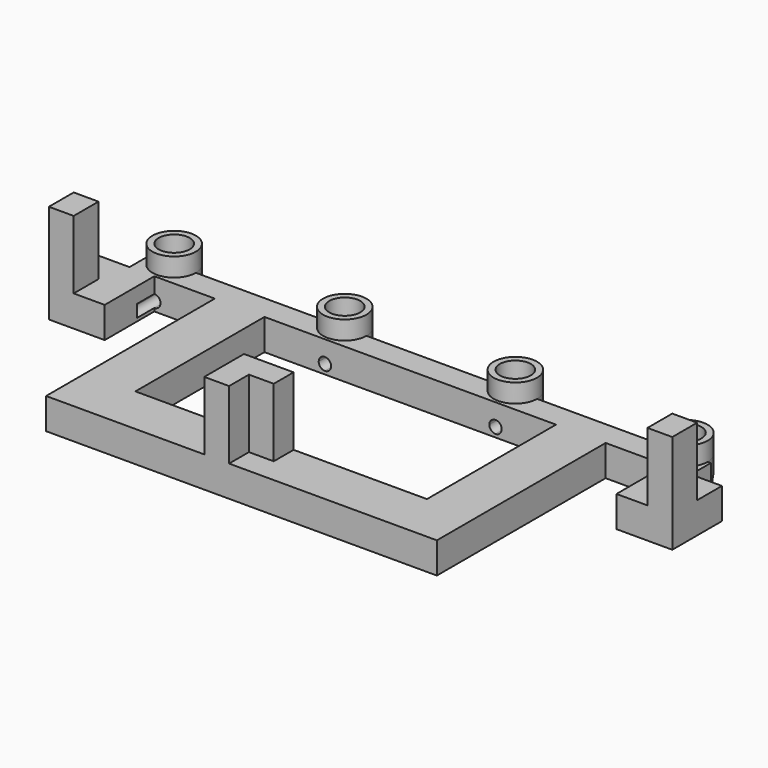
from build123d import *

# Parameters (mm, degrees)
F0_W         = 4
F0_H         = 26
F0_W_2       = 2
F0_H_2       = 4
F0_H_3       = 5
F1_DEPTH     = 5
F2_DEPTH     = 16
F3_R         = 3.5
F3_R_2       = 2.5
F4_DEPTH     = 3
F6_DEPTH     = 7.5
F7_T4_DEPTH  = 26.8255996257
F7_S5_R      = 3.5
F7_T6_DEPTH  = 15
F7_S7_R      = 2.5
F7_T8_DEPTH  = 15
F7_T12_DEPTH = 26.8255996257
F7_S13_R     = 3.5
F7_T14_DEPTH = 15
F7_S15_R     = 2.5
F7_T16_DEPTH = 15
F7_T20_DEPTH = 26.8255996257
F7_S21_R     = 3.5
F7_T22_DEPTH = 15
F7_S23_R     = 2.5
F7_T24_DEPTH = 15
F7_T28_DEPTH = 26.8255996257
F7_S29_R     = 3.5
F7_T30_DEPTH = 15
F7_S31_R     = 2.5
F7_T32_DEPTH = 15
F7_T36_DEPTH = 26.8255996257
F7_S37_R     = 3.5
F7_T38_DEPTH = 15
F7_S39_R     = 2.5
F7_T40_DEPTH = 15
F7_T44_DEPTH = 26.8255996257
F7_S45_R     = 3.5
F7_T46_DEPTH = 15
F7_S47_R     = 2.5
F7_T48_DEPTH = 15
F7_T52_DEPTH = 26.8255996257
F7_S53_R     = 3.5
F7_T54_DEPTH = 15
F7_S55_R     = 2.5
F7_T56_DEPTH = 15
F7_T60_DEPTH = 26.8255996257
F7_S61_R     = 3.5
F7_T62_DEPTH = 15
F7_S63_R     = 2.5
F7_T64_DEPTH = 15


# Not quite as in the source:
# - a fillet or chamfer that OpenCascade refuses, or shapes differently, is made with other operations: its cross-section is extruded or revolved along the edge and cut away or added


with BuildPart() as f1:
    # F0 (on Top) → F1 (new body)
    with BuildSketch(Plane.XY):
        with BuildLine():
            ThreePointArc((27.5, -4), (24.6715728753, -2.8284271247), (23.5, 0))
            Line((23.5, 0), (17.75, 0))
            Line((17.75, 0), (17.75, -4))
            Line((17.75, -4), (27.5, -4))
        make_face()
        with Locations((15.75, -17)):
            Rectangle(F0_W, F0_H)
        with BuildLine():
            Line((52.5, 0), (51, 0))
            ThreePointArc((51, 0), (52.1715728753, -2.8284271247), (55, -4))
            Line((55, -4), (55, -2.5))
            ThreePointArc((55, -2.5), (53.232233047, -1.767766953), (52.5, 0))
        make_face()
        with Locations((42.25, -32)):
            Rectangle(F0_W_2, F0_H_2)
        with BuildLine():
            ThreePointArc((82.5, -2.5), (84.267766953, -1.767766953), (85, 0))
            Line((85, 0), (82.5, 0))
            Line((82.5, 0), (82.5, -2.5))
        make_face()
        with BuildLine():
            Line((82.5, 0), (80, 0))
            ThreePointArc((80, 0), (80.732233047, -1.767766953), (82.5, -2.5))
            Line((82.5, -2.5), (82.5, 0))
        make_face()
        Polygon((47.25, -38), (47.25, -30), (43.25, -30), (43.25, -34), (43.25, -38), align=None)
        with BuildLine():
            Line((64.75, 0), (59, 0))
            ThreePointArc((59, 0), (57.8284271247, -2.8284271247), (55, -4))
            Line((55, -4), (64.75, -4))
            Line((64.75, -4), (64.75, 0))
        make_face()
        with Locations((11.75, -2)):
            Rectangle(F0_W, F0_H_2)
        with Locations((42.25, -36)):
            Rectangle(F0_W_2, F0_H_2)
        with Locations((40.25, -32)):
            Rectangle(F0_W_2, F0_H_2)
        with Locations((11.75, -17)):
            Rectangle(F0_W, F0_H)
        with Locations((70.75, -2)):
            Rectangle(F0_W, F0_H_2)
        with BuildLine():
            Line((25, 0), (23.5, 0))
            ThreePointArc((23.5, 0), (24.6715728753, -2.8284271247), (27.5, -4))
            Line((27.5, -4), (27.5, -2.5))
            ThreePointArc((27.5, -2.5), (25.732233047, -1.767766953), (25, 0))
        make_face()
        with Locations((40.25, -36)):
            Rectangle(F0_W_2, F0_H_2)
        Polygon((35.25, -30), (35.25, -38), (39.25, -38), (39.25, -34), (39.25, -30), align=None)
        with BuildLine():
            ThreePointArc((55, -4), (57.8284271247, -2.8284271247), (59, 0))
            Line((59, 0), (57.5, 0))
            ThreePointArc((57.5, 0), (56.767766953, -1.767766953), (55, -2.5))
            Line((55, -2.5), (55, -4))
        make_face()
        with Locations((70.75, -17)):
            Rectangle(F0_W, F0_H)
        with Locations((66.75, -2)):
            Rectangle(F0_W, F0_H_2)
        with BuildLine():
            Line((55, 0), (52.5, 0))
            ThreePointArc((52.5, 0), (53.232233047, -1.767766953), (55, -2.5))
            Line((55, -2.5), (55, 0))
        make_face()
        with BuildLine():
            Line((0, -4), (0, -2.5))
            ThreePointArc((0, -2.5), (-1.767766953, -1.767766953), (-2.5, 0))
            Line((-2.5, 0), (-4, 0))
            ThreePointArc((-4, 0), (-2.8284271247, -2.8284271247), (0, -4))
        make_face()
        Polygon((86.5, -4), (82.5, -4), (82.5, -14), (87.5, -14), (87.5, -9), (87.5, -4), align=None)
        with BuildLine():
            Line((-4, -4), (0, -4))
            ThreePointArc((0, -4), (-2.8284271247, -2.8284271247), (-4, 0))
            Line((-4, 0), (-4, -4))
        make_face()
        with BuildLine():
            Line((86.5, -4), (86.5, 0))
            ThreePointArc((86.5, 0), (85.3284271247, -2.8284271247), (82.5, -4))
            Line((82.5, -4), (86.5, -4))
        make_face()
        with Locations((-7, -6.5)):
            Rectangle(F0_W, F0_H_3)
        with Locations((89.5, -6.5)):
            Rectangle(F0_W, F0_H_3)
        with Locations((-7, -11.5)):
            Rectangle(F0_W, F0_H_3)
        with Locations((89.5, -11.5)):
            Rectangle(F0_W, F0_H_3)
        with BuildLine():
            Line((2.5, 0), (0, 0))
            Line((0, 0), (0, -2.5))
            ThreePointArc((0, -2.5), (1.767766953, -1.767766953), (2.5, 0))
        make_face()
        with BuildLine():
            Line((9.75, 0), (4, 0))
            ThreePointArc((4, 0), (2.8284271247, -2.8284271247), (0, -4))
            Line((0, -4), (9.75, -4))
            Line((9.75, -4), (9.75, 0))
        make_face()
        with BuildLine():
            Line((27.5, 0), (25, 0))
            ThreePointArc((25, 0), (25.732233047, -1.767766953), (27.5, -2.5))
            Line((27.5, -2.5), (27.5, 0))
        make_face()
        with BuildLine():
            ThreePointArc((27.5, -2.5), (29.267766953, -1.767766953), (30, 0))
            Line((30, 0), (27.5, 0))
            Line((27.5, 0), (27.5, -2.5))
        make_face()
        with Locations((66.75, -17)):
            Rectangle(F0_W, F0_H)
        with BuildLine():
            ThreePointArc((27.5, -4), (30.3284271247, -2.8284271247), (31.5, 0))
            Line((31.5, 0), (30, 0))
            ThreePointArc((30, 0), (29.267766953, -1.767766953), (27.5, -2.5))
            Line((27.5, -2.5), (27.5, -4))
        make_face()
        with BuildLine():
            Line((0, -2.5), (0, 0))
            Line((0, 0), (-2.5, 0))
            ThreePointArc((-2.5, 0), (-1.767766953, -1.767766953), (0, -2.5))
        make_face()
        with BuildLine():
            ThreePointArc((55, -2.5), (56.767766953, -1.767766953), (57.5, 0))
            Line((57.5, 0), (55, 0))
            Line((55, 0), (55, -2.5))
        make_face()
        with BuildLine():
            ThreePointArc((82.5, -4), (85.3284271247, -2.8284271247), (86.5, 0))
            Line((86.5, 0), (85, 0))
            ThreePointArc((85, 0), (84.267766953, -1.767766953), (82.5, -2.5))
            Line((82.5, -2.5), (82.5, -4))
        make_face()
        Polygon((13.75, -30), (9.75, -30), (9.75, -38), (35.25, -38), (35.25, -30), (17.75, -30), align=None)
        with BuildLine():
            Line((51, 0), (31.5, 0))
            ThreePointArc((31.5, 0), (30.3284271247, -2.8284271247), (27.5, -4))
            Line((27.5, -4), (55, -4))
            ThreePointArc((55, -4), (52.1715728753, -2.8284271247), (51, 0))
        make_face()
        with BuildLine():
            ThreePointArc((82.5, -4), (79.6715728753, -2.8284271247), (78.5, 0))
            Line((78.5, 0), (72.75, 0))
            Line((72.75, 0), (72.75, -4))
            Line((72.75, -4), (82.5, -4))
        make_face()
        with Locations((15.75, -2)):
            Rectangle(F0_W, F0_H_2)
        with BuildLine():
            Line((4, 0), (2.5, 0))
            ThreePointArc((2.5, 0), (1.767766953, -1.767766953), (0, -2.5))
            Line((0, -2.5), (0, -4))
            ThreePointArc((0, -4), (2.8284271247, -2.8284271247), (4, 0))
        make_face()
        Polygon((68.75, -30), (64.75, -30), (47.25, -30), (47.25, -38), (72.75, -38), (72.75, -30), align=None)
        Polygon((0, -14), (0, -4), (-4, -4), (-5, -4), (-5, -9), (-5, -14), align=None)
        with BuildLine():
            Line((80, 0), (78.5, 0))
            ThreePointArc((78.5, 0), (79.6715728753, -2.8284271247), (82.5, -4))
            Line((82.5, -4), (82.5, -2.5))
            ThreePointArc((82.5, -2.5), (80.732233047, -1.767766953), (80, 0))
        make_face()
    extrude(amount=F1_DEPTH)

    # F0 (on Top) → F2 (join)
    with BuildSketch(Plane.XY):
        with Locations((-7, -11.5)):
            Rectangle(F0_W, F0_H_3)
        with Locations((89.5, -11.5)):
            Rectangle(F0_W, F0_H_3)
        Polygon((35.25, -30), (35.25, -38), (39.25, -38), (39.25, -34), (39.25, -30), align=None)
        with Locations((40.25, -32)):
            Rectangle(F0_W_2, F0_H_2)
        with Locations((42.25, -32)):
            Rectangle(F0_W_2, F0_H_2)
    extrude(amount=F2_DEPTH)

    # F3 (on face) → F4 (join)
    with BuildSketch(Plane.XY.offset(5)):
        Circle(F3_R)
        Circle(F3_R_2, mode=Mode.SUBTRACT)
        with BuildLine():
            ThreePointArc((86, 0), (82.5, 3.5), (79, 0))
            ThreePointArc((79, 0), (82.5, -3.5), (86, 0))
        make_face()
        with BuildLine():
            ThreePointArc((85, 0), (82.5, -2.5), (80, 0))
            ThreePointArc((80, 0), (82.5, 2.5), (85, 0))
        make_face(mode=Mode.SUBTRACT)
        with BuildLine():
            ThreePointArc((58.5, 0), (55, 3.5), (51.5, 0))
            Line((51.5, 0), (52.5, 0))
            ThreePointArc((52.5, 0), (55, 2.5), (57.5, 0))
            Line((57.5, 0), (58.5, 0))
        make_face()
        with BuildLine():
            Line((52.5, 0), (51.5, 0))
            ThreePointArc((51.5, 0), (55, -3.5), (58.5, 0))
            Line((58.5, 0), (57.5, 0))
            ThreePointArc((57.5, 0), (55, -2.5), (52.5, 0))
        make_face()
        with BuildLine():
            ThreePointArc((31, 0), (27.5, 3.5), (24, 0))
            Line((24, 0), (25, 0))
            ThreePointArc((25, 0), (27.5, 2.5), (30, 0))
            Line((30, 0), (31, 0))
        make_face()
        with BuildLine():
            Line((25, 0), (24, 0))
            ThreePointArc((24, 0), (27.5, -3.5), (31, 0))
            Line((31, 0), (30, 0))
            ThreePointArc((30, 0), (27.5, -2.5), (25, 0))
        make_face()
    extrude(amount=F4_DEPTH)

    # F5 (on face) → F6 (cut)
    with BuildSketch(Plane(origin=(0, 0, 0), x_dir=(-1, 0, 0), z_dir=(0, 1, 0))):
        with BuildLine():
            ThreePointArc((0, 2.5), (-1, 1.5), (0, 0.5))
            Line((0, 0.5), (0, 2.5))
        make_face()
        with BuildLine():
            Line((0, 2.5), (0, 0.5))
            ThreePointArc((0, 0.5), (0.7071067812, 0.7928932188), (1, 1.5))
            ThreePointArc((1, 1.5), (0.7071067812, 2.2071067812), (0, 2.5))
        make_face()
        with BuildLine():
            ThreePointArc((-82.5, 2.5), (-83.5, 1.5), (-82.5, 0.5))
            Line((-82.5, 0.5), (-82.5, 2.5))
        make_face()
        with BuildLine():
            Line((-82.5, 2.5), (-82.5, 0.5))
            ThreePointArc((-82.5, 0.5), (-81.7928932188, 0.7928932188), (-81.5, 1.5))
            ThreePointArc((-81.5, 1.5), (-81.7928932188, 2.2071067812), (-82.5, 2.5))
        make_face()
        with BuildLine():
            ThreePointArc((-55, 2.5), (-56, 1.5), (-55, 0.5))
            Line((-55, 0.5), (-55, 2.5))
        make_face()
        with BuildLine():
            Line((-55, 2.5), (-55, 0.5))
            ThreePointArc((-55, 0.5), (-54.2928932188, 0.7928932188), (-54, 1.5))
            ThreePointArc((-54, 1.5), (-54.2928932188, 2.2071067812), (-55, 2.5))
        make_face()
        with BuildLine():
            ThreePointArc((-27.5, 2.5), (-28.5, 1.5), (-27.5, 0.5))
            Line((-27.5, 0.5), (-27.5, 2.5))
        make_face()
        with BuildLine():
            Line((-27.5, 2.5), (-27.5, 0.5))
            ThreePointArc((-27.5, 0.5), (-26.7928932188, 0.7928932188), (-26.5, 1.5))
            ThreePointArc((-26.5, 1.5), (-26.7928932188, 2.2071067812), (-27.5, 2.5))
        make_face()
    extrude(amount=-F6_DEPTH, mode=Mode.SUBTRACT)

    # F7: chamfer of 5 x 3.5 on 8 edges, made by hand


with BuildPart() as f7_tool2:
    # F7_s3 → F7_t4 (new body)
    with BuildSketch(Plane.YZ.offset(16.4127998128)):
        Polygon((0, 0), (3.5, 5), (0, 5), align=None)
    extrude(amount=-F7_T4_DEPTH)

    # F7_s5 → F7_t6 (intersect, symmetric)
    with BuildSketch(Plane.XY.offset(2.5)):
        Circle(F7_S5_R)
    extrude(amount=F7_T6_DEPTH, both=True, mode=Mode.INTERSECT)

    # F7_s7 → F7_t8 (cut, symmetric)
    with BuildSketch(Plane.XY.offset(2.5)):
        Circle(F7_S7_R)
    extrude(amount=F7_T8_DEPTH, both=True, mode=Mode.SUBTRACT)


with BuildPart() as f1_1:
    add(f1.part)

    # F7_t1: union F7_tool2
    add(f7_tool2.part)


with BuildPart() as f7_tool10:
    # F7_s11 → F7_t12 (new body)
    with BuildSketch(Plane.YZ.offset(37.9127998128)):
        Polygon((0, 0), (3.5, 5), (0, 5), align=None)
    extrude(amount=-F7_T12_DEPTH)

    # F7_s13 → F7_t14 (intersect, symmetric)
    with BuildSketch(Plane.XY.offset(2.5)):
        with Locations((27.5, 0)):
            Circle(F7_S13_R)
    extrude(amount=F7_T14_DEPTH, both=True, mode=Mode.INTERSECT)

    # F7_s15 → F7_t16 (cut, symmetric)
    with BuildSketch(Plane.XY.offset(2.5)):
        with Locations((27.5, 0)):
            Circle(F7_S15_R)
    extrude(amount=F7_T16_DEPTH, both=True, mode=Mode.SUBTRACT)


with BuildPart() as f1_2:
    add(f1_1.part)

    # F7_t9: union F7_tool10
    add(f7_tool10.part)


with BuildPart() as f7_tool18:
    # F7_s19 → F7_t20 (new body)
    with BuildSketch(Plane.YZ.offset(65.4127998128)):
        Polygon((0, 0), (3.5, 5), (0, 5), align=None)
    extrude(amount=-F7_T20_DEPTH)

    # F7_s21 → F7_t22 (intersect, symmetric)
    with BuildSketch(Plane.XY.offset(2.5)):
        with Locations((55, 0)):
            Circle(F7_S21_R)
    extrude(amount=F7_T22_DEPTH, both=True, mode=Mode.INTERSECT)

    # F7_s23 → F7_t24 (cut, symmetric)
    with BuildSketch(Plane.XY.offset(2.5)):
        with Locations((55, 0)):
            Circle(F7_S23_R)
    extrude(amount=F7_T24_DEPTH, both=True, mode=Mode.SUBTRACT)


with BuildPart() as f1_3:
    add(f1_2.part)

    # F7_t17: union F7_tool18
    add(f7_tool18.part)


with BuildPart() as f7_tool26:
    # F7_s27 → F7_t28 (new body)
    with BuildSketch(Plane.YZ.offset(43.9127998128)):
        Polygon((0, 0), (3.5, 5), (0, 5), align=None)
    extrude(amount=-F7_T28_DEPTH)

    # F7_s29 → F7_t30 (intersect, symmetric)
    with BuildSketch(Plane.XY.offset(2.5)):
        with Locations((27.5, 0)):
            Circle(F7_S29_R)
    extrude(amount=F7_T30_DEPTH, both=True, mode=Mode.INTERSECT)

    # F7_s31 → F7_t32 (cut, symmetric)
    with BuildSketch(Plane.XY.offset(2.5)):
        with Locations((27.5, 0)):
            Circle(F7_S31_R)
    extrude(amount=F7_T32_DEPTH, both=True, mode=Mode.SUBTRACT)


with BuildPart() as f1_4:
    add(f1_3.part)

    # F7_t25: union F7_tool26
    add(f7_tool26.part)


with BuildPart() as f7_tool34:
    # F7_s35 → F7_t36 (new body)
    with BuildSketch(Plane.YZ.offset(92.9127998128)):
        Polygon((0, 0), (3.5, 5), (0, 5), align=None)
    extrude(amount=-F7_T36_DEPTH)

    # F7_s37 → F7_t38 (intersect, symmetric)
    with BuildSketch(Plane.XY.offset(2.5)):
        with Locations((82.5, 0)):
            Circle(F7_S37_R)
    extrude(amount=F7_T38_DEPTH, both=True, mode=Mode.INTERSECT)

    # F7_s39 → F7_t40 (cut, symmetric)
    with BuildSketch(Plane.XY.offset(2.5)):
        with Locations((82.5, 0)):
            Circle(F7_S39_R)
    extrude(amount=F7_T40_DEPTH, both=True, mode=Mode.SUBTRACT)


with BuildPart() as f1_5:
    add(f1_4.part)

    # F7_t33: union F7_tool34
    add(f7_tool34.part)


with BuildPart() as f7_tool42:
    # F7_s43 → F7_t44 (new body)
    with BuildSketch(Plane.YZ.offset(71.4127998128)):
        Polygon((0, 0), (3.5, 5), (0, 5), align=None)
    extrude(amount=-F7_T44_DEPTH)

    # F7_s45 → F7_t46 (intersect, symmetric)
    with BuildSketch(Plane.XY.offset(2.5)):
        with Locations((55, 0)):
            Circle(F7_S45_R)
    extrude(amount=F7_T46_DEPTH, both=True, mode=Mode.INTERSECT)

    # F7_s47 → F7_t48 (cut, symmetric)
    with BuildSketch(Plane.XY.offset(2.5)):
        with Locations((55, 0)):
            Circle(F7_S47_R)
    extrude(amount=F7_T48_DEPTH, both=True, mode=Mode.SUBTRACT)


with BuildPart() as f1_6:
    add(f1_5.part)

    # F7_t41: union F7_tool42
    add(f7_tool42.part)


with BuildPart() as f7_tool50:
    # F7_s51 → F7_t52 (new body)
    with BuildSketch(Plane.YZ.offset(10.4127998128)):
        Polygon((0, 0), (3.5, 5), (0, 5), align=None)
    extrude(amount=-F7_T52_DEPTH)

    # F7_s53 → F7_t54 (intersect, symmetric)
    with BuildSketch(Plane.XY.offset(2.5)):
        Circle(F7_S53_R)
    extrude(amount=F7_T54_DEPTH, both=True, mode=Mode.INTERSECT)

    # F7_s55 → F7_t56 (cut, symmetric)
    with BuildSketch(Plane.XY.offset(2.5)):
        Circle(F7_S55_R)
    extrude(amount=F7_T56_DEPTH, both=True, mode=Mode.SUBTRACT)


with BuildPart() as f1_7:
    add(f1_6.part)

    # F7_t49: union F7_tool50
    add(f7_tool50.part)


with BuildPart() as f7_tool58:
    # F7_s59 → F7_t60 (new body)
    with BuildSketch(Plane.YZ.offset(98.9127998128)):
        Polygon((0, 0), (3.5, 5), (0, 5), align=None)
    extrude(amount=-F7_T60_DEPTH)

    # F7_s61 → F7_t62 (intersect, symmetric)
    with BuildSketch(Plane.XY.offset(2.5)):
        with Locations((82.5, 0)):
            Circle(F7_S61_R)
    extrude(amount=F7_T62_DEPTH, both=True, mode=Mode.INTERSECT)

    # F7_s63 → F7_t64 (cut, symmetric)
    with BuildSketch(Plane.XY.offset(2.5)):
        with Locations((82.5, 0)):
            Circle(F7_S63_R)
    extrude(amount=F7_T64_DEPTH, both=True, mode=Mode.SUBTRACT)


with BuildPart() as f1_8:
    add(f1_7.part)

    # F7_t57: union F7_tool58
    add(f7_tool58.part)


solid = f1_8.part
